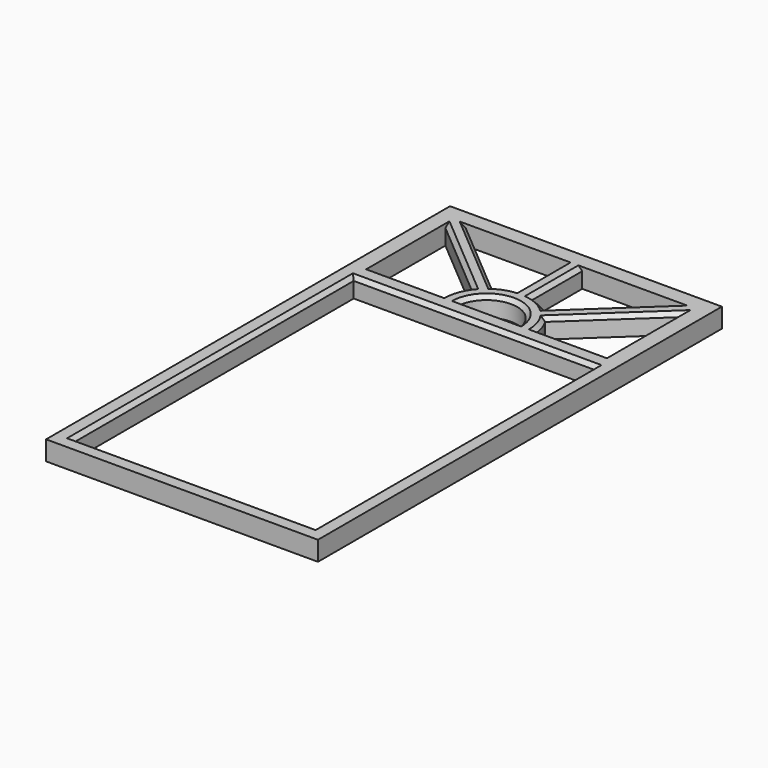
from build123d import *

# Parameters (mm, degrees)
F0_W     = 700
F0_H     = 1300
F0_W_2   = 620
F0_H_2   = 900
F1_DEPTH = 50
F2_SIZE  = 10


# Not quite as in the source:
# - a feature names something its author has since deleted; it is built from what else it names


with BuildPart() as f1:
    # F0 (on Top) → F1 (new body)
    with BuildSketch(Plane.XY):
        with Locations((-12.4809433535, 115.0203361814)):
            Rectangle(F0_W, F0_H)
        with Locations((-12.4809433535, -44.9796638186)):
            Rectangle(F0_W_2, F0_H_2, mode=Mode.SUBTRACT)
        Polygon((-131.3545905658, 445.0203361814), (-322.4809433535, 445.0203361814), (-322.4809433535, 700.0203361814), (-322.4809433535, 725.0203361814), (-290.108913989, 725.0203361814), (-30.108913989, 725.0203361814), (9.891086011, 725.0203361814), (265.6861508147, 725.0203361814), (297.5190566465, 725.0203361814), (297.5190566465, 700.0203361814), (297.5190566465, 445.0203361814), (106.3927038589, 445.0203361814), (66.3927038589, 445.0203361814), (-91.3545905658, 445.0203361814), align=None, mode=Mode.SUBTRACT)
        with BuildLine():
            Line((-322.4809433535, 725.0203361814), (-322.4809433535, 700.0203361814))
            Line((-322.4809433535, 700.0203361814), (-106.829258799, 517.3345075045))
            ThreePointArc((-106.829258799, 517.3345075045), (-93.2073200284, 532.2796973439), (-77.2493518889, 544.6998087791))
            Line((-77.2493518889, 544.6998087791), (-290.108913989, 725.0203361814))
            Line((-290.108913989, 725.0203361814), (-322.4809433535, 725.0203361814))
        make_face()
        with BuildLine():
            ThreePointArc((-106.829258799, 517.3345075045), (-125.0564121886, 483.2002761775), (-131.3545905658, 445.0203361814))
            Line((-131.3545905658, 445.0203361814), (-91.3545905658, 445.0203361814))
            ThreePointArc((-91.3545905658, 445.0203361814), (-12.4809433535, 523.8939833937), (66.3927038589, 445.0203361814))
            Line((66.3927038589, 445.0203361814), (106.3927038589, 445.0203361814))
            ThreePointArc((106.3927038589, 445.0203361814), (102.1362449296, 476.5456300205), (89.6716866284, 505.8132978575))
            ThreePointArc((89.6716866284, 505.8132978575), (77.9737439548, 522.1494068715), (63.691579675, 536.2819970091))
            ThreePointArc((63.691579675, 536.2819970091), (38.4127121689, 552.4483578012), (9.891086011, 561.7697957248))
            ThreePointArc((9.891086011, 561.7697957248), (-10.0745975152, 563.8696252044), (-30.108913989, 562.5796771664))
            ThreePointArc((-30.108913989, 562.5796771664), (-54.6379504639, 556.16767422), (-77.2493518889, 544.6998087791))
            ThreePointArc((-77.2493518889, 544.6998087791), (-93.2073200284, 532.2796973439), (-106.829258799, 517.3345075045))
        make_face()
        with BuildLine():
            Line((-30.108913989, 725.0203361814), (-30.108913989, 562.5796771664))
            ThreePointArc((-30.108913989, 562.5796771664), (-10.0745975152, 563.8696252044), (9.891086011, 561.7697957248))
            Line((9.891086011, 561.7697957248), (9.891086011, 725.0203361814))
            Line((9.891086011, 725.0203361814), (-30.108913989, 725.0203361814))
        make_face()
        with BuildLine():
            ThreePointArc((63.691579675, 536.2819970091), (77.9737439548, 522.1494068715), (89.6716866284, 505.8132978575))
            Line((89.6716866284, 505.8132978575), (297.5190566465, 700.0203361814))
            Line((297.5190566465, 700.0203361814), (297.5190566465, 725.0203361814))
            Line((297.5190566465, 725.0203361814), (265.6861508147, 725.0203361814))
            Line((265.6861508147, 725.0203361814), (63.691579675, 536.2819970091))
        make_face()
    extrude(amount=F1_DEPTH)

    # F2
    f2_edges = [f1.edges().sort_by_distance(p)[0] for p in [
        (-12.480943, 405.020336, 50),
        (297.519057, -44.979664, 50),
        (-12.480943, -494.979664, 50),
        (-322.480943, -44.979664, 50),
        (-12.480943, 523.893983, 50),
        (-54.63795, 556.167674, 50),
        (102.136245, 476.54563, 50),
        (-214.655101, 608.677422, 50),
        (-183.679133, 634.860072, 50),
        (-30.108914, 643.800007, 50),
        (38.412712, 552.448358, 50),
        (-125.056412, 483.200276, 50),
        (193.595372, 602.916817, 50),
        (164.688865, 630.651167, 50),
        (9.891086, 643.395066, 50),
    ]]
    chamfer(f2_edges, length=F2_SIZE)


solid = f1.part
